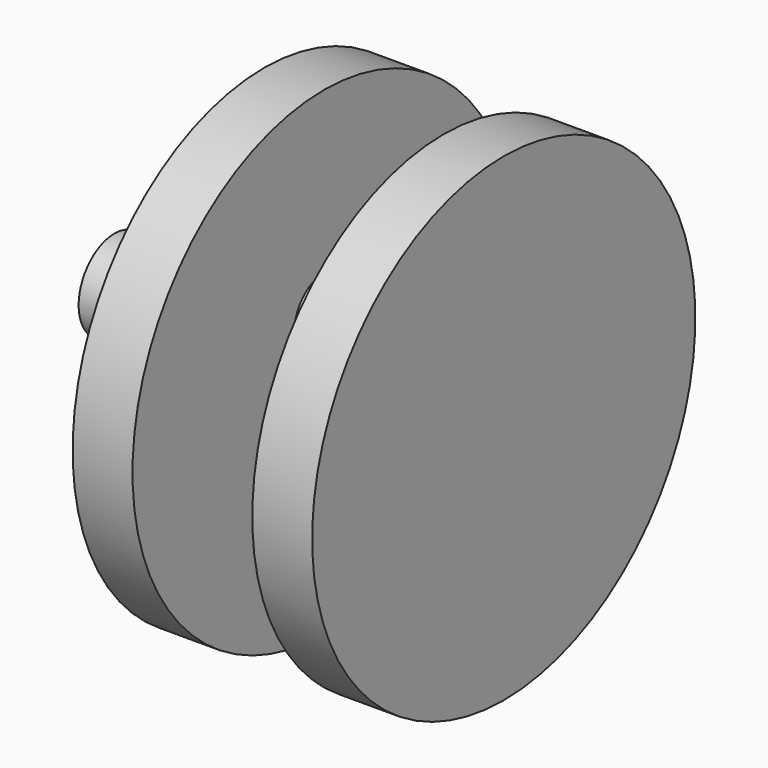
from build123d import *

# Parameters (mm, degrees)
F0_W = 31.75
F0_H = 9.525
F2_W = 25.4
F2_H = 7.9375


# Not quite as in the source:
# - a feature names something its author has since deleted; it is built from what else it names


with BuildPart() as f1:
    # F0 (on Front) → F1 (revolve)
    with BuildSketch(Plane.XZ):
        with Locations((-41.275, 4.7625)):
            Rectangle(F0_W, F0_H)
        Polygon((-25.4, 9.525), (-25.4, 0), (-12.7, 0), (-12.7, 38.89375), (-12.7, 46.83125), (-12.7, 50.8), (-25.4, 50.8), align=None)
    revolve(axis=Axis((-41.275, 0, 0), (-1, 0, 0)))



with BuildPart() as f1b:
    # F0 (on Front) → F1, piece 2 (revolve)
    with BuildSketch(Plane.XZ):
        Polygon((12.7, 46.83125), (12.7, 38.89375), (12.7, 0), (25.4, 0), (25.4, 9.525), (25.4, 50.8), (12.7, 50.8), align=None)
    revolve(axis=Axis((-41.275, 0, 0), (-1, 0, 0)))


with BuildPart() as f1_1:
    add(f1.part)

    add(f1b.part)  # F3 merges F1b
    # F2 (on Front) → F3 (revolve)
    with BuildSketch(Plane.XZ):
        with Locations((0, 12.7)):
            Rectangle(F2_W, F2_H)
    revolve(axis=Axis((0, 0, 8.73125), (1, 0, 0)))


solid = f1_1.part
